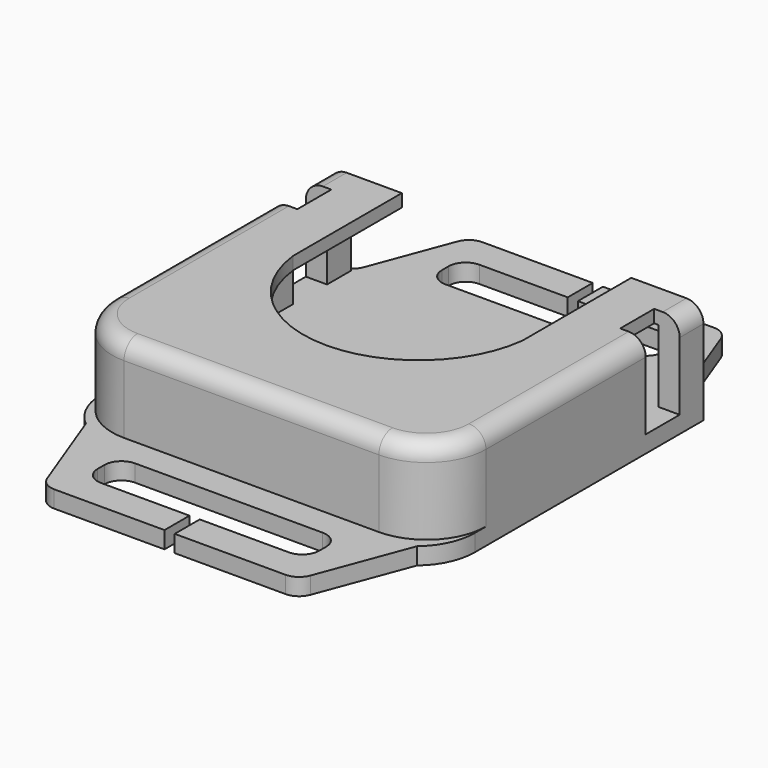
from build123d import *

# Parameters (mm, degrees)
F1_DEPTH     = 8.5
F0_W         = 39
F0_H         = 36.5
F2_DEPTH     = 1.5
F3_W         = 44
F3_H         = 39
F4_DEPTH     = 1.5
F6_DEPTH     = 2
F7_W         = 3
F7_H         = 5
F8_DEPTH     = 10
F9_R         = 7
F10_R        = 2
F0_W_2       = 26.0822549462
F0_H_2       = 5
F11_DEPTH    = 2
F12_T1_DEPTH = 28.8095132369
F13_R        = 2
F14_R        = 2
F15_W        = 1.200100407
F15_H        = 3.7374552339
F16_DEPTH    = 5


# Not quite as in the source:
# - a fillet or chamfer that OpenCascade refuses, or shapes differently, is made with other operations: its cross-section is extruded or revolved along the edge and cut away or added


with BuildPart() as f1:
    # F0 (on Top) → F1 (new body)
    with BuildSketch(Plane.XY):
        Polygon((22, -19.5), (22, 19.5), (19.5, 19.5), (19.5, -17), (-19.5, -17), (-19.5, 19.5), (-22, 19.5), (-22, -19.5), (-19.5, -19.5), (19.5, -19.5), align=None)
    extrude(amount=F1_DEPTH)

    # F0 (on Top) → F2 (join)
    with BuildSketch(Plane.XY):
        with Locations((0, 1.25)):
            Rectangle(F0_W, F0_H)
        Polygon((22, -19.5), (22, 19.5), (19.5, 19.5), (19.5, -17), (-19.5, -17), (-19.5, 19.5), (-22, 19.5), (-22, -19.5), (-19.5, -19.5), (19.5, -19.5), align=None)
    extrude(amount=-F2_DEPTH)

    # F3 (on face) → F4 (join)
    with BuildSketch(Plane.XY.offset(8.5)):
        Rectangle(F3_W, F3_H)
    extrude(amount=F4_DEPTH)

    # F5 (on face) → F6 (cut)
    with BuildSketch(Plane.XY.offset(10)):
        with BuildLine():
            Line((13.5, 3.5), (13.5, 19.5))
            Line((13.5, 19.5), (-13.5, 19.5))
            Line((-13.5, 19.5), (-13.5, 3.5))
            ThreePointArc((-13.5, 3.5), (0, -8.5), (13.5, 3.5))
        make_face()
    extrude(amount=-F6_DEPTH, mode=Mode.SUBTRACT)

    # F7 (on face) → F8 (cut)
    with BuildSketch(Plane.XY.offset(10)):
        with Locations((20.5, 13.5)):
            Rectangle(F7_W, F7_H)
        with Locations((-20.5, 13.5)):
            Rectangle(F7_W, F7_H)
    extrude(amount=-F8_DEPTH, mode=Mode.SUBTRACT)

    # F9
    f9_edges = [f1.edges().sort_by_distance(p)[0] for p in [
        (22, -19.5, 4.25),
        (-22, -19.5, 4.25),
    ]]
    fillet(f9_edges, radius=F9_R)

    # F10
    f10_edges = [f1.edges().sort_by_distance(p)[0] for p in [
        (-22, -0.75, 10),
        (-22, 17.75, 10),
        (-19.949747, -17.449747, 10),
        (0, -19.5, 10),
        (19.949747, -17.449747, 10),
        (22, -0.75, 10),
        (22, 17.75, 10),
    ]]
    fillet(f10_edges, radius=F10_R)

    # F0 (on Top) → F11 (join)
    with BuildSketch(Plane.XY):
        Polygon((22, -19.5), (22, 19.5), (19.5, 19.5), (19.5, -17), (-19.5, -17), (-19.5, 19.5), (-22, 19.5), (-22, -19.5), (-19.5, -19.5), (19.5, -19.5), align=None)
        with Locations((0, 1.25)):
            Rectangle(F0_W, F0_H)
        Polygon((-19.5, 19.5), (19.5, 19.5), (15, 31.5), (-15, 31.5), align=None)
        with Locations((0, 25.3217592835)):
            Rectangle(F0_W_2, F0_H_2, mode=Mode.SUBTRACT)
        Polygon((15, -31.5), (19.5, -19.5), (-19.5, -19.5), (-15, -31.5), align=None)
        with Locations((0, -25.3217592835)):
            Rectangle(F0_W_2, F0_H_2, mode=Mode.SUBTRACT)
    extrude(amount=-F11_DEPTH)

    # F12: fillet of radius 7 on 2 edges, made by hand

    # F12_s2 → F12_t1 (cut)
    with BuildSketch(Plane.XY.offset(-15.4047566185)):
        with BuildLine():
            ThreePointArc((-22, -14.1380973526), (-21.3442887702, -17.0961372442), (-19.5, -19.5))
            Line((-19.5, -19.5), (-19.59, -19.6072380529))
            ThreePointArc((-19.59, -19.6072380529), (-20.75, -19.64), (-22, -19.64))
            Line((-22, -19.64), (-22.14, -19.5))
            Line((-22.14, -19.5), (-22.14, -14.1380973526))
            Line((-22.14, -14.1380973526), (-22, -14.1380973526))
        make_face()
        with BuildLine():
            ThreePointArc((22, -14.1380973526), (21.3442887702, -17.0961372442), (19.5, -19.5))
            Line((19.5, -19.5), (19.59, -19.6072380529))
            ThreePointArc((19.59, -19.6072380529), (20.75, -19.64), (22, -19.64))
            Line((22, -19.64), (22.14, -19.5))
            Line((22.14, -19.5), (22.14, -14.1380973526))
            Line((22.14, -14.1380973526), (22, -14.1380973526))
        make_face()
    extrude(amount=F12_T1_DEPTH, mode=Mode.SUBTRACT)

    # F13
    f13_edges = [f1.edges().sort_by_distance(p)[0] for p in [
        (15, 31.5, -1),
        (19.5, 19.5, -1),
        (-19.5, 19.5, -1),
        (-15, 31.5, -1),
        (15, -31.5, -1),
        (-15, -31.5, -1),
    ]]
    fillet(f13_edges, radius=F13_R)

    # F14
    f14_edges = [f1.edges().sort_by_distance(p)[0] for p in [
        (-13.041127, 22.821759, -1),
        (-13.041127, 27.821759, -1),
        (13.041127, 27.821759, -1),
        (13.041127, 22.821759, -1),
        (13.041127, -27.821759, -1),
        (13.041127, -22.821759, -1),
        (-13.041127, -22.821759, -1),
        (-13.041127, -27.821759, -1),
    ]]
    fillet(f14_edges, radius=F14_R)

    # F15 (on face) → F16 (cut)
    with BuildSketch(Plane.XY):
        with Locations((-0.0326880836, 29.6578230336)):
            Rectangle(F15_W, F15_H)
        with Locations((-0.0326880836, -29.6578230336)):
            Rectangle(F15_W, F15_H)
    extrude(amount=-F16_DEPTH, mode=Mode.SUBTRACT)


solid = f1.part
